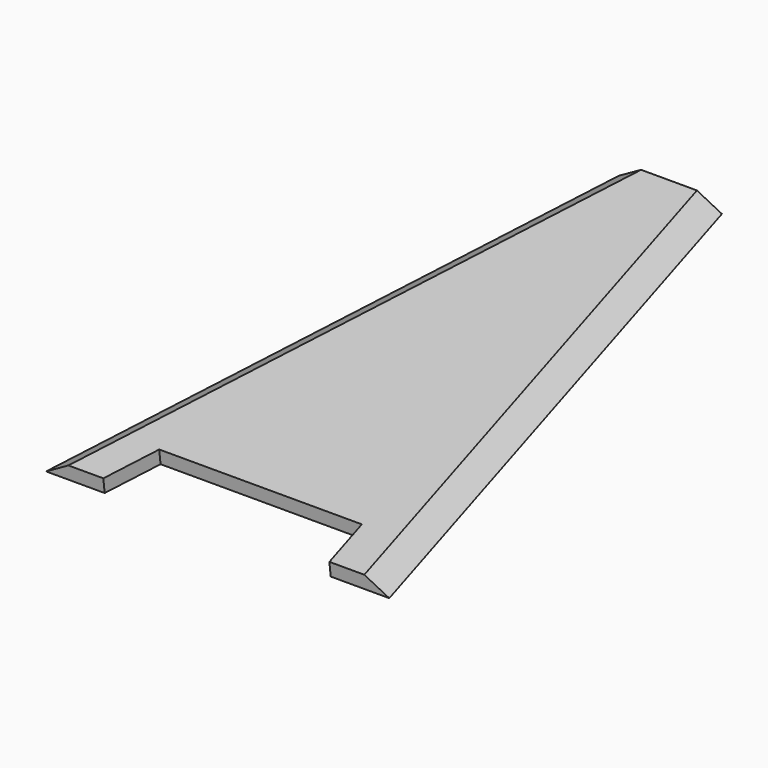
from build123d import *

# Parameters (mm, degrees)
F7_R      = 411.1162199172
F8_DEPTH  = 245.8819093104
F10_DEPTH = 72.1732122579
F13_R     = 303.0795059163
F14_DEPTH = 62.9709492631
F16_R     = 347.3761175619
F17_DEPTH = 62.9709492631
F18_W     = 90
F18_H     = 35.3622667967
F19_DEPTH = 72.1732122579
F20_W     = 378.0467361212
F20_H     = 51.6974163429
F21_DEPTH = 72.1732122579


with BuildPart() as f5:
    # F1 (on Front) → F5 section 0
    with BuildSketch(Plane.XZ):
        Polygon((-150, -86.6025403784), (150, -86.6025403784), (0, 173.2050807569), align=None)
    # F4 (on line) → F5 section 1
    with BuildSketch(Plane(origin=(0, 495, 0), x_dir=(-1, 0, 0), z_dir=(0, 1, 0))):
        Polygon((-45, -25.9807621135), (45, -25.9807621135), (0, 51.9615242271), align=None)
    loft()

    # F7 (on face) → F8 (cut, through all)
    with BuildSketch(Plane(origin=(0, 8.9906162556, -73.4118195457), x_dir=(1, 0, 0), z_dir=(0, 0.1215600245, -0.9925840823))):
        with Locations((0, -288.0104482174)):
            Circle(F7_R)
    extrude(amount=-F8_DEPTH, mode=Mode.SUBTRACT)

    # F9 (on face) → F10 (cut, through all)
    with BuildSketch(Plane(origin=(0, 10.4493365501, -85.3228285333), x_dir=(1, 0, 0), z_dir=(0, 0.1215600245, -0.9925840823))):
        Polygon((88.3763476395, -39.4725930665), (98.9037545729, 10.5274069335), (-98.9037545729, 10.5274069335), (-88.3763476395, -39.4725930665), align=None)
    extrude(amount=-F10_DEPTH, mode=Mode.SUBTRACT)

    # F13 (on face) → F14 (cut, through all)
    with BuildSketch(Plane(origin=(0, 0, 0), x_dir=(0.8660254038, 0, 0.5), z_dir=(0.5, 0, -0.8660254038))):
        with Locations((-100.1057326794, -240.2520924807)):
            Circle(F13_R)
    extrude(amount=-F14_DEPTH, mode=Mode.SUBTRACT)

    # F16 (on face) → F17 (cut, through all)
    with BuildSketch(Plane(origin=(0, 0, 0), x_dir=(0.8660254038, 0, -0.5), z_dir=(-0.5, 0, -0.8660254038))):
        with Locations((93.3309048414, -267.9739892483)):
            Circle(F16_R)
    extrude(amount=-F17_DEPTH, mode=Mode.SUBTRACT)

    # F18 (on face) → F19 (cut, through all)
    with BuildSketch(Plane(origin=(0, 10.4493365501, -85.3228285333), x_dir=(1, 0, 0), z_dir=(0, 0.1215600245, -0.9925840823))):
        with Locations((0, -505.8520320565)):
            Rectangle(F18_W, F18_H)
    extrude(amount=-F19_DEPTH, mode=Mode.SUBTRACT)

    # F20 (on face) → F21 (cut, through all)
    with BuildSketch(Plane(origin=(0, 8.9906162556, -73.4118195457), x_dir=(1, 0, 0), z_dir=(0, -0.1215600245, 0.9925840823))):
        with Locations((11.1420080066, -34.9064962379)):
            Rectangle(F20_W, F20_H)
    extrude(amount=-F21_DEPTH, mode=Mode.SUBTRACT)


solid = f5.part
